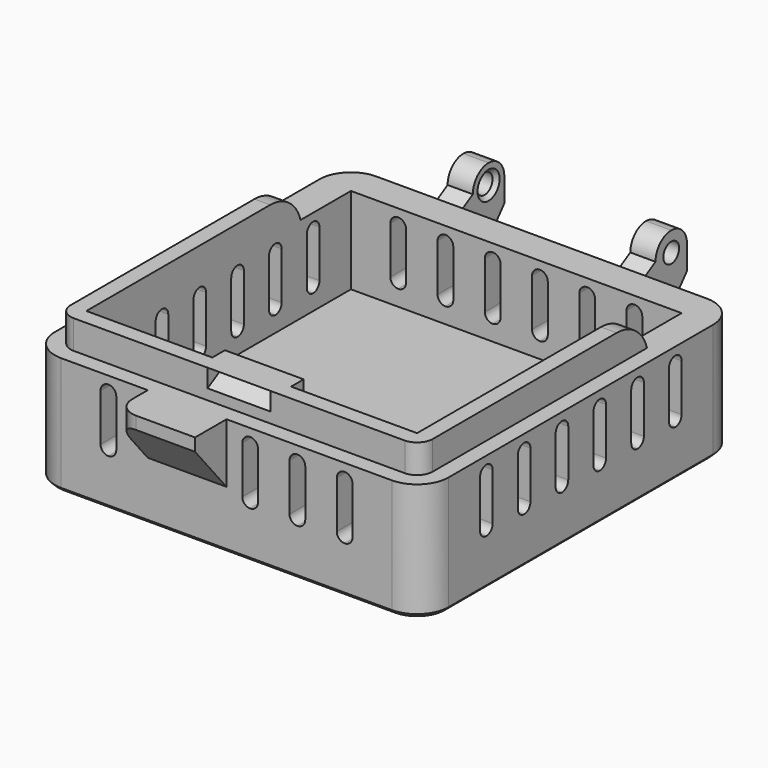
from build123d import *

# Parameters (mm, degrees)
F0_W         = 50
F0_H         = 50
F1_DEPTH     = 20
F2_T         = -4
F3_R         = 4
F5_DEPTH     = 50
F7_DEPTH     = 50.001
F8_W         = 50
F8_H         = 50
F8_W_2       = 46
F8_H_2       = 46
F9_DEPTH     = 5
F10_T1_DEPTH = 10.0024143135
F12_DEPTH    = 5
F14_DEPTH    = 4
F15_W        = 46
F15_H        = 46
F16_DEPTH    = 1.35
F17_W        = 46
F17_H        = 10
F18_DEPTH    = 25
F19_T1_DEPTH = 26.0715080541
F19_T3_DEPTH = 26.0715080541
F21_R        = 1.25
F22_DEPTH    = 3.2
F23_R        = 2.49999
F24_W        = 12
F24_H        = 15
F25_DEPTH    = 4
F27_DEPTH    = 10
F28_SIZE     = 0.5
F30_R        = 2.49999


# Not quite as in the source:
# - a fillet or chamfer that OpenCascade refuses, or shapes differently, is made with other operations: its cross-section is extruded or revolved along the edge and cut away or added
# - two fillets or chamfers of one size are made in one step
# - a fillet or chamfer is up to 0.001 mm smaller than in the source, because OpenCascade refuses the exact size
# - a pattern or mirror of a feature is missing from the dataset's text; its kind, count and spacing are read off the source's solid


with BuildPart() as f1:
    # F0 (on Top) → F1 (new body)
    with BuildSketch(Plane.XY):
        Rectangle(F0_W, F0_H)
    extrude(amount=F1_DEPTH)

    # F2
    f2_openings = [f1.faces().sort_by_distance(p)[0] for p in [
        (0, 0, 20),
    ]]
    offset(amount=F2_T, openings=f2_openings)

    # F3
    f3_edges = [f1.edges().sort_by_distance(p)[0] for p in [
        (-25, -25, 10),
        (25, -25, 10),
        (25, 25, 10),
        (-25, 25, 10),
    ]]
    fillet(f3_edges, radius=F3_R)

    # F4 (on face) → F5 (cut)
    with BuildSketch(Plane.XZ.offset(25)):
        with BuildLine():
            ThreePointArc((-15, 6), (-14.2928932188, 6.2928932188), (-14, 7))
            Line((-14, 7), (-14, 13))
            ThreePointArc((-14, 13), (-14.2928932188, 13.7071067812), (-15, 14))
            ThreePointArc((-15, 14), (-15.7071067812, 13.7071067812), (-16, 13))
            Line((-16, 13), (-16, 7))
            ThreePointArc((-16, 7), (-15.7071067812, 6.2928932188), (-15, 6))
        make_face()
        with BuildLine():
            Line((-10, 13), (-10, 7))
            ThreePointArc((-10, 7), (-9.7071067812, 6.2928932188), (-9, 6))
            ThreePointArc((-9, 6), (-8.2928932188, 6.2928932188), (-8, 7))
            Line((-8, 7), (-8, 13))
            ThreePointArc((-8, 13), (-8.2928932188, 13.7071067812), (-9, 14))
            ThreePointArc((-9, 14), (-9.7071067812, 13.7071067812), (-10, 13))
        make_face()
        with BuildLine():
            Line((-4, 13), (-4, 7))
            ThreePointArc((-4, 7), (-3.7071067812, 6.2928932188), (-3, 6))
            ThreePointArc((-3, 6), (-2.2928932188, 6.2928932188), (-2, 7))
            Line((-2, 7), (-2, 13))
            ThreePointArc((-2, 13), (-2.2928932188, 13.7071067812), (-3, 14))
            ThreePointArc((-3, 14), (-3.7071067812, 13.7071067812), (-4, 13))
        make_face()
        with BuildLine():
            Line((2, 13), (2, 7))
            ThreePointArc((2, 7), (2.2928932188, 6.2928932188), (3, 6))
            ThreePointArc((3, 6), (3.7071067812, 6.2928932188), (4, 7))
            Line((4, 7), (4, 13))
            ThreePointArc((4, 13), (3.7071067812, 13.7071067812), (3, 14))
            ThreePointArc((3, 14), (2.2928932188, 13.7071067812), (2, 13))
        make_face()
        with BuildLine():
            Line((8, 13), (8, 7))
            ThreePointArc((8, 7), (8.2928932188, 6.2928932188), (9, 6))
            ThreePointArc((9, 6), (9.7071067812, 6.2928932188), (10, 7))
            Line((10, 7), (10, 13))
            ThreePointArc((10, 13), (9.7071067812, 13.7071067812), (9, 14))
            ThreePointArc((9, 14), (8.2928932188, 13.7071067812), (8, 13))
        make_face()
        with BuildLine():
            ThreePointArc((15, 6), (15.7071067812, 6.2928932188), (16, 7))
            Line((16, 7), (16, 13))
            ThreePointArc((16, 13), (15.7071067812, 13.7071067812), (15, 14))
            ThreePointArc((15, 14), (14.2928932188, 13.7071067812), (14, 13))
            Line((14, 13), (14, 7))
            ThreePointArc((14, 7), (14.2928932188, 6.2928932188), (15, 6))
        make_face()
    extrude(amount=-F5_DEPTH, mode=Mode.SUBTRACT)

    # F6 (on face) → F7 (cut, through all)
    with BuildSketch(Plane.YZ.offset(25)):
        with BuildLine():
            ThreePointArc((-15, 6), (-14.2928932188, 6.2928932188), (-14, 7))
            Line((-14, 7), (-14, 13))
            ThreePointArc((-14, 13), (-14.2928932188, 13.7071067812), (-15, 14))
            ThreePointArc((-15, 14), (-15.7071067812, 13.7071067812), (-16, 13))
            Line((-16, 13), (-16, 7))
            ThreePointArc((-16, 7), (-15.7071067812, 6.2928932188), (-15, 6))
        make_face()
        with BuildLine():
            Line((-10, 13), (-10, 7))
            ThreePointArc((-10, 7), (-9.7071067812, 6.2928932188), (-9, 6))
            ThreePointArc((-9, 6), (-8.2928932188, 6.2928932188), (-8, 7))
            Line((-8, 7), (-8, 13))
            ThreePointArc((-8, 13), (-8.2928932188, 13.7071067812), (-9, 14))
            ThreePointArc((-9, 14), (-9.7071067812, 13.7071067812), (-10, 13))
        make_face()
        with BuildLine():
            Line((-4, 13), (-4, 7))
            ThreePointArc((-4, 7), (-3.7071067812, 6.2928932188), (-3, 6))
            ThreePointArc((-3, 6), (-2.2928932188, 6.2928932188), (-2, 7))
            Line((-2, 7), (-2, 13))
            ThreePointArc((-2, 13), (-2.2928932188, 13.7071067812), (-3, 14))
            ThreePointArc((-3, 14), (-3.7071067812, 13.7071067812), (-4, 13))
        make_face()
        with BuildLine():
            ThreePointArc((9, 6), (9.7071067812, 6.2928932188), (10, 7))
            Line((10, 7), (10, 13))
            ThreePointArc((10, 13), (9.7071067812, 13.7071067812), (9, 14))
            ThreePointArc((9, 14), (8.2928932188, 13.7071067812), (8, 13))
            Line((8, 13), (8, 7))
            ThreePointArc((8, 7), (8.2928932188, 6.2928932188), (9, 6))
        make_face()
        with BuildLine():
            ThreePointArc((15, 6), (15.7071067812, 6.2928932188), (16, 7))
            Line((16, 7), (16, 13))
            ThreePointArc((16, 13), (15.7071067812, 13.7071067812), (15, 14))
            ThreePointArc((15, 14), (14.2928932188, 13.7071067812), (14, 13))
            Line((14, 13), (14, 7))
            ThreePointArc((14, 7), (14.2928932188, 6.2928932188), (15, 6))
        make_face()
        with BuildLine():
            ThreePointArc((3, 14), (2.2928932188, 13.7071067812), (2, 13))
            Line((2, 13), (2, 7))
            ThreePointArc((2, 7), (2.2928932188, 6.2928932188), (3, 6))
            ThreePointArc((3, 6), (3.7071067812, 6.2928932188), (4, 7))
            Line((4, 7), (4, 13))
            ThreePointArc((4, 13), (3.7071067812, 13.7071067812), (3, 14))
        make_face()
    extrude(amount=-F7_DEPTH, mode=Mode.SUBTRACT)

    # F8 (on face) → F9 (cut)
    with BuildSketch(Plane.XY.offset(20)):
        Rectangle(F8_W, F8_H)
        Rectangle(F8_W_2, F8_H_2, mode=Mode.SUBTRACT)
    extrude(amount=-F9_DEPTH, mode=Mode.SUBTRACT)

    # F10: fillet of radius 2 on 3 edges, made by hand

    # F10_s2 → F10_t1 (cut)
    with BuildSketch(Plane.XY.offset(15)):
        with BuildLine():
            ThreePointArc((-20.9990343146, 23.0004), (-22.4142135624, 22.4142135624), (-23.0004, 20.9990343146))
            Line((-23.0004, 20.9990343146), (-23.2005365685, 20.9990343146))
            ThreePointArc((-23.2005365685, 20.9990343146), (-23.2001365685, 21.9995171573), (-23.2001365685, 23))
            Line((-23.2001365685, 23), (-23, 23.2001365685))
            ThreePointArc((-23, 23.2001365685), (-21.9995171573, 23.2001365685), (-20.9990343146, 23.2005365685))
            Line((-20.9990343146, 23.2005365685), (-20.9990343146, 23.0004))
        make_face()
        with BuildLine():
            ThreePointArc((-23.0004, -20.9990343146), (-22.4142135624, -22.4142135624), (-20.9990343146, -23.0004))
            Line((-20.9990343146, -23.0004), (-20.9990343146, -23.2005365685))
            ThreePointArc((-20.9990343146, -23.2005365685), (-21.9995171573, -23.2001365685), (-23, -23.2001365685))
            Line((-23, -23.2001365685), (-23.2001365685, -23))
            ThreePointArc((-23.2001365685, -23), (-23.2001365685, -21.9995171573), (-23.2005365685, -20.9990343146))
            Line((-23.2005365685, -20.9990343146), (-23.0004, -20.9990343146))
        make_face()
        with BuildLine():
            ThreePointArc((23.0004, -20.9990343146), (22.4142135624, -22.4142135624), (20.9990343146, -23.0004))
            Line((20.9990343146, -23.0004), (20.9990343146, -23.2005365685))
            ThreePointArc((20.9990343146, -23.2005365685), (21.9995171573, -23.2001365685), (23, -23.2001365685))
            Line((23, -23.2001365685), (23.2001365685, -23))
            ThreePointArc((23.2001365685, -23), (23.2001365685, -21.9995171573), (23.2005365685, -20.9990343146))
            Line((23.2005365685, -20.9990343146), (23.0004, -20.9990343146))
        make_face()
    extrude(amount=F10_T1_DEPTH, mode=Mode.SUBTRACT)

    # F11 (on Right) → F12 (join, symmetric)
    with BuildSketch(Plane.YZ):
        Polygon((-19, 18.8452994616), (-21, 20), (-21, 15), (-19, 16.1547005384), align=None)
    extrude(amount=F12_DEPTH, both=True)

    # F13 (on Right) → F14 (cut, symmetric)
    with BuildSketch(Plane.YZ):
        Polygon((-21, 17.5), (-23, 18.6547005384), (-23, 16.3452994616), align=None)
    extrude(amount=F14_DEPTH, both=True, mode=Mode.SUBTRACT)

    # F15 (on face) → F16 (cut)
    with BuildSketch(Plane.XY.offset(20)):
        Rectangle(F15_W, F15_H)
    extrude(amount=-F16_DEPTH, mode=Mode.SUBTRACT)

    # F17 (on face) → F18 (cut)
    with BuildSketch(Plane.XY.offset(15)):
        with Locations((0, 18)):
            Rectangle(F17_W, F17_H)
    extrude(amount=F18_DEPTH, mode=Mode.SUBTRACT)

    # F19: fillet of radius 5 on 2 edges, made by hand

    # F19_s2 → F19_t1 (cut)
    with BuildSketch(Plane.YZ.offset(-35.0357540271)):
        with BuildLine():
            ThreePointArc((8.1856983892, 18.65), (11.2064598826, 17.6343443626), (13, 15))
            Line((13, 15), (13, 18.65))
            Line((13, 18.65), (8.1856983892, 18.65))
        make_face()
    extrude(amount=F19_T1_DEPTH, mode=Mode.SUBTRACT)

    # F19_s4 → F19_t3 (cut)
    with BuildSketch(Plane.YZ.offset(8.9642459729)):
        with BuildLine():
            ThreePointArc((8.1856983892, 18.65), (11.2064598826, 17.6343443626), (13, 15))
            Line((13, 15), (13, 18.65))
            Line((13, 18.65), (8.1856983892, 18.65))
        make_face()
    extrude(amount=F19_T3_DEPTH, mode=Mode.SUBTRACT)

    # F21 (on offset) → F22 (join)
    with BuildSketch(Plane.YZ.offset(10)):
        Polygon((26.6, 15.9237604307), (25, 15), (25, 5), (31.6, 12.8655737111), (31.6, 18.4237604307), (26.6, 18.4237604307), align=None)
        with Locations((29.1, 15.9237604307)):
            Circle(F21_R, mode=Mode.SUBTRACT)
    f22 = extrude(amount=F22_DEPTH)

    # F22_copies: F22 across plane
    add(f22.mirror(Plane(origin=(0, 0, 0), x_dir=(0, 0, -1), z_dir=(-1, 0, 0))))

    # F23 (radius 2.5 in the source; OpenCascade refuses exactly that, so slightly less here)
    f23_edges = [f1.edges().sort_by_distance(p)[0] for p in [
        (11.6, 26.6, 18.42376),
        (11.6, 31.6, 18.42376),
    ]]
    fillet(f23_edges, radius=F23_R)

    # F24 (on face) → F25 (join)
    with BuildSketch(Plane.XZ.offset(25)):
        with Locations((-6, 7.5)):
            Rectangle(F24_W, F24_H)
    extrude(amount=-F25_DEPTH)

    # F26 (on Right) → F27 (join)
    with BuildSketch(Plane.YZ):
        Polygon((-25, 7.441232037), (-25, 15), (-30, 15), (-30, 13.4), align=None)
    extrude(amount=-F27_DEPTH)

    # F28
    f28_edges = [f1.edges().sort_by_distance(p)[0] for p in [
        (10, 27.85, 15.92376),
        (0, 25, 0),
        (-23.828427, -23.828427, 0),
        (0, -25, 0),
        (23.828427, -23.828427, 0),
        (25, 0, 0),
        (23.828427, 23.828427, 0),
        (-23.828427, 23.828427, 0),
        (-25, 0, 0),
        (-10, 27.85, 15.92376),
    ]]
    chamfer(f28_edges, length=F28_SIZE)

    # F30 (radius 2.5 in the source; OpenCascade refuses exactly that, so slightly less here)
    f30_edges = [f1.edges().sort_by_distance(p)[0] for p in [
        (-10, -30, 14.2),
        (-11.6, 31.6, 18.42376),
        (-11.6, 26.6, 18.42376),
    ]]
    fillet(f30_edges, radius=F30_R)


solid = f1.part
